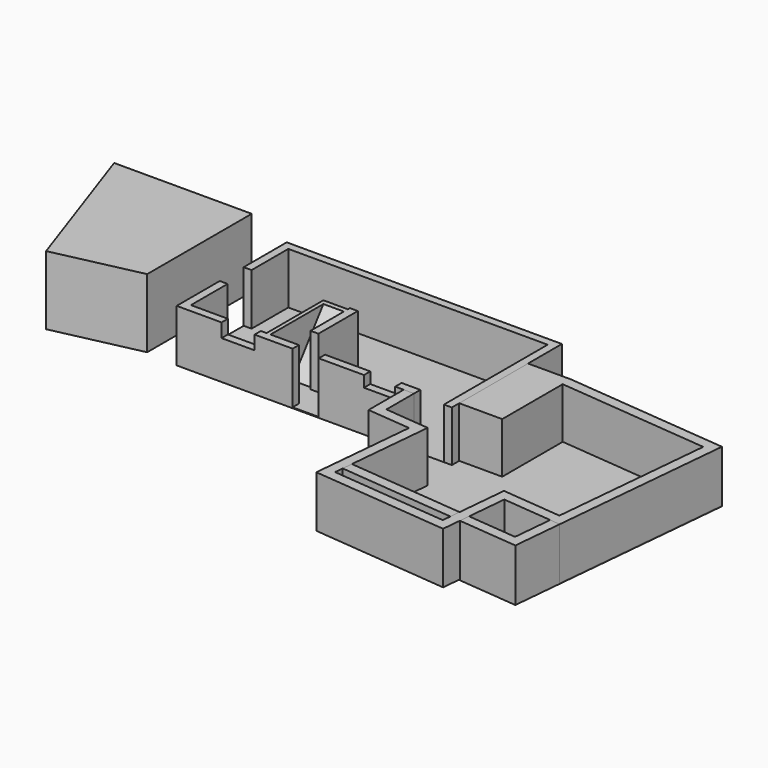
from build123d import *

# Parameters (mm, degrees)
F4_DEPTH  = 1500
F5_DEPTH  = 1500
F3_W      = 230
F3_H      = 1430
F6_W      = 760
F6_H      = 1500
F6_W_2    = 910
F6_H_2    = 325
F6_W_3    = 960
F6_H_3    = 402
F7_DEPTH  = 230
F8_DEPTH  = 25
F10_DEPTH = 25
F12_DEPTH = 115
F14_DEPTH = 595
F15_W     = 870
F15_H     = 1500
F16_DEPTH = 230
F18_DEPTH = 25
F20_DEPTH = 1500
F22_DEPTH = 2000


with BuildPart() as f4:
    # F2 (on Top) → F4 (new body)
    with BuildSketch(Plane.XY):
        Polygon((9250, 269), (9250, 2467.6854490471), (13666.3567495496, 2053.7978043052), (13092.5117789977, -4069.3714690182), (7964.9797858895, -3588.8346237594), (8196.0522462423, -1123.1934458246), (6900, -1001.7313352933), (6900, 0), (6600, 0), (6600, -1274.9307903732), (7869.3686245898, -1393.8921923013), (7638.296164237, -3859.533370236), (13363.2105254744, -4396.0550906707), (13993.040371202, 2324.4965507819), (9250, 2769), (8000, 2769), (8000, 269), align=None)
    extrude(amount=F4_DEPTH)

    # F1 (on Top) → F10 (join)
    with BuildSketch(Plane.XY):
        Polygon((13993.040371202, 2324.4965507819), (9250, 2769), (8000, 2769), (8000, 0), (6600, 0), (6600, -1274.9307903732), (7869.3686245898, -1393.8921923013), (7638.296164237, -3859.533370236), (13363.2105254744, -4396.0550906707), align=None)
    extrude(amount=-F10_DEPTH)


with BuildPart() as f5:
    # F3 (on Top) → F5 (new body)
    with BuildSketch(Plane.XY):
        Polygon((8000, 4000), (0, 4000), (0, 0), (6900, 0), (6900, 230), (2545, 230), (2545, 1170), (2430, 1170), (2430, 230), (230, 230), (230, 3770), (7770, 3770), (7770, 0), (8000, 0), (8000, 269), (8000, 2769), (8000, 3790), align=None)
    extrude(amount=F5_DEPTH)

    # F6 (on face) → F7 (cut, through all)
    with BuildSketch(Plane.XZ):
        with Locations((3750, 750)):
            Rectangle(F6_W, F6_H)
        with Locations((5900, 1337.5)):
            Rectangle(F6_W_2, F6_H_2)
        with Locations((1785, 1299)):
            Rectangle(F6_W_3, F6_H_3)
    extrude(amount=-F7_DEPTH, mode=Mode.SUBTRACT)



with BuildPart() as f5b:
    # F3 (on Top) → F5, piece 2 (new body)
    with BuildSketch(Plane.XY):
        with Locations((3255, 1655)):
            Rectangle(F3_W, F3_H)
    extrude(amount=F5_DEPTH)


with BuildPart() as f5_1:
    add(f5.part)

    add(f5b.part)  # F8 merges F5b
    # F0 (on Top) → F8 (join)
    with BuildSketch(Plane.XY):
        Polygon((0, 4000), (0, 0), (8000, 0), (8000, 269), (8000, 2769), (8000, 3790), (8000, 4000), align=None)
    extrude(amount=-F8_DEPTH)

    # F9: union 

    # F11 (on face) → F12 (join, through all)
    with BuildSketch(Plane(origin=(2430, 0, 0), x_dir=(0, -1, 0), z_dir=(-1, 0, 0))):
        Polygon((-2295, 1500), (-1170, 0), (-1170, 1500), align=None)
    extrude(amount=-F12_DEPTH)

    # F13 (on face) → F14 (join, through all)
    with BuildSketch(Plane.YZ.offset(2545)):
        Polygon((1170, 0), (2295, 1500), (2151.25, 1500), (1026.25, 0), align=None)
    extrude(amount=F14_DEPTH)

    # F15 (on face) → F16 (cut)
    with BuildSketch(Plane(origin=(0, 0, 0), x_dir=(0, -1, 0), z_dir=(-1, 0, 0))):
        with Locations((-2000, 750)):
            Rectangle(F15_W, F15_H)
    extrude(amount=-F16_DEPTH, mode=Mode.SUBTRACT)


with BuildPart() as f18:
    # F17 (on Top) → F18 (new body)
    with BuildSketch(Plane.XY):
        Polygon((13993.0403712021, 2324.4965507819), (9250, 2769), (8000, 2769), (8000, 269), (8000, 0), (6600, 0), (6600, -1274.9307903732), (7869.3686245898, -1393.8921923013), (7586.9766953259, -4407.1338743544), (11569.5258161867, -4780.3663755263), (11756.1420667726, -2789.0918150959), (13498.5073071492, -2952.3810343586), align=None)
    extrude(amount=F18_DEPTH)


with BuildPart() as f20:
    # F19 (on Top) → F20 (new body)
    with BuildSketch(Plane.XY):
        Polygon((6900, -1001.7313352933), (6900, 0), (6600, 0), (6600, -1274.9307903732), (7869.3686245898, -1393.8921923013), (7586.9766953259, -4407.1338743544), (11569.5258161867, -4780.3663755263), (11756.1420667726, -2789.0918150959), (13498.5073071492, -2952.3810343586), (13993.0403712021, 2324.4965507819), (9250, 2769), (8000, 2769), (8000, 269), (9250, 269), (9250, 2467.6854490471), (13666.3567495496, 2053.7978043052), (13227.8085606726, -2625.6974127062), (11485.443320296, -2462.4081934435), (11298.82706971, -4453.6827538739), (7913.6603169784, -4136.4351278777), (8196.0522462423, -1123.1934458246), align=None)
    extrude(amount=F20_DEPTH)


with BuildPart() as f22:
    # F21 (on Top) → F22 (new body)
    with BuildSketch(Plane.XY):
        Polygon((-3396.867229657, -499.8484626007), (-896.867229657, 48.7145184311), (-896.867229657, 3848.7145184311), (-4896.867229657, 3848.7145184311), align=None)
    extrude(amount=F22_DEPTH)


solid = Compound([f4.part, f5_1.part, f18.part, f20.part, f22.part])
